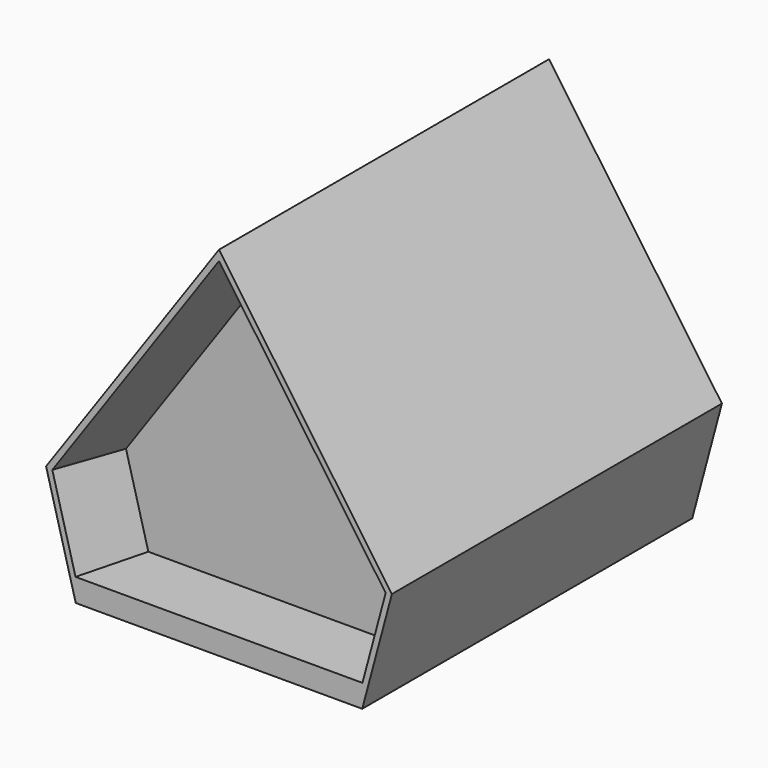
from build123d import *

# Parameters (mm, degrees)
F1_DEPTH = 3600
F2_T     = -200
F3_DEPTH = 3000
F4_SIZE2 = 599.99999
F4_SIZE  = 149.99999
F6_DEPTH = 100


# Not quite as in the source:
# - a fillet or chamfer is up to 0.001 mm smaller than in the source, because OpenCascade refuses the exact size


with BuildPart() as f1:
    # F0 (on Front) → F1 (new body)
    with BuildSketch(Plane.XZ):
        Polygon((1508.8190451025, 965.9258262891), (0, 3120.7427380868), (-1508.8190451025, 965.9258262891), (-1250, 0), (0, 0), (1250, 0), align=None)
    extrude(amount=-F1_DEPTH)

    # F2
    f2_openings = [f1.faces().sort_by_distance(p)[0] for p in [
        (0, 0, 1149.918376),
    ]]
    offset(amount=F2_T, openings=f2_openings)

    # F3 (add): a face of the model
    f3_faces = [f1.faces().sort_by_distance(p)[0] for p in [
        (0, 3600, 1149.9183758236),
    ]]
    extrude(f3_faces, amount=-F3_DEPTH)

    # F4 (size 150 and 600 in the source; OpenCascade refuses exactly that, so slightly less here)
    f4_edges = [f1.edges().sort_by_distance(p)[0] for p in [
        (-1194.015311, 0, 563.802957),
        (-645.74801, 0, 1849.829646),
        (645.74801, 0, 1849.829646),
        (1194.015311, 0, 563.802957),
    ]]
    f4_side = f1.faces().sort_by_distance((718.849289, 0, 2018.434739))[0]
    chamfer(f4_edges, length=F4_SIZE, length2=F4_SIZE2, reference=f4_side)

    # F5 (on face) → F6 (cut)
    with BuildSketch(Plane(origin=(0, 3600, 0), x_dir=(-1, 0, 0), z_dir=(0, 1, 0))):
        Polygon((0, 2772.0533789626), (-1291.4960192832, 927.6059133079), (-1096.5346024042, 200), (1096.5346024042, 200), (1291.4960192832, 927.6059133079), align=None)
    extrude(amount=-F6_DEPTH, mode=Mode.SUBTRACT)


solid = f1.part
